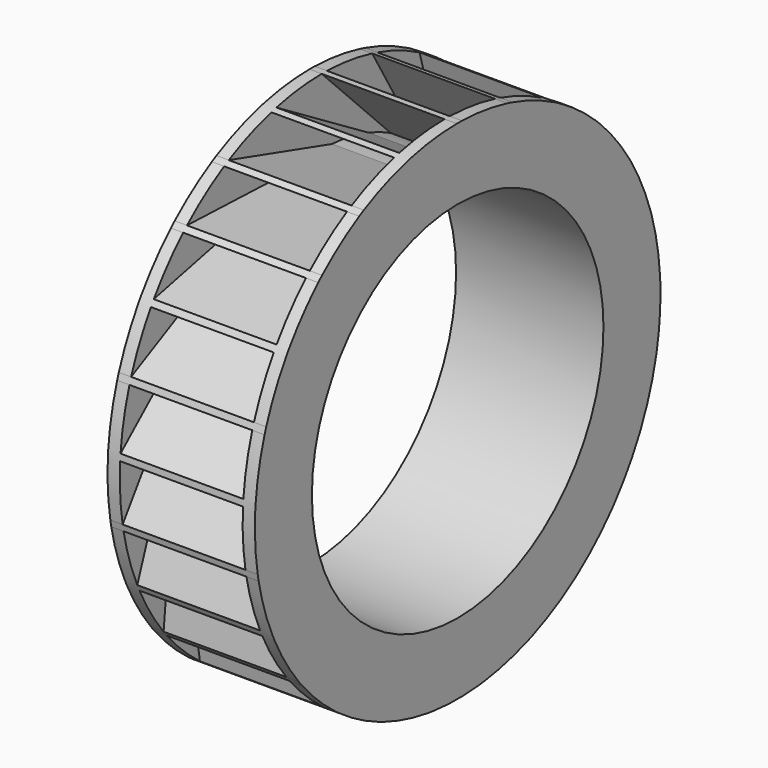
from build123d import *

# Parameters (mm, degrees)
F1_DEPTH      = 44
F1_DEPTH_BACK = 4
F2_DEPTH      = 40


with BuildPart() as f1:
    # F0 (on Right) → F1 (new body, two sides)
    with BuildSketch(Plane.YZ) as f1_sk:
        with BuildLine():
            Line((47.9947331255, -37.3985428132), (81.1532544526, -15.1212364493))
            ThreePointArc((81.1532544526, -15.1212364493), (82.2000719436, -7.5928039926), (82.55, 0))
            ThreePointArc((82.55, 0), (82.5323765572, 1.7056728359), (82.4795137535, 3.41061739))
            Line((82.4795137535, 3.41061739), (53.3191059714, -29.3124265585))
            ThreePointArc((53.3191059714, -29.3124265585), (50.81800682, -33.4615539863), (47.9947331255, -37.3985428132))
        make_face()
        with BuildLine():
            ThreePointArc((80.7364542136, -17.2083543957), (80.9515809502, -16.166138737), (81.1532544526, -15.1212364493))
            Line((81.1532544526, -15.1212364493), (47.9947331255, -37.3985428132))
            ThreePointArc((47.9947331255, -37.3985428132), (46.2234468965, -39.5668847567), (44.354284157, -41.6514452242))
            Line((44.354284157, -41.6514452242), (80.7364542136, -17.2083543957))
        make_face()
        with BuildLine():
            ThreePointArc((74.8431771472, -34.8281686931), (78.2870991132, -26.1845873071), (80.7364542136, -17.2083543957))
            Line((80.7364542136, -17.2083543957), (44.354284157, -41.6514452242))
            ThreePointArc((44.354284157, -41.6514452242), (40.8999156028, -45.0482221184), (37.1862509359, -48.1594035851))
            Line((37.1862509359, -48.1594035851), (74.8431771472, -34.8281686931))
        make_face()
        with BuildLine():
            ThreePointArc((44.354284157, -41.6514452242), (46.2234468965, -39.5668847567), (47.9947331255, -37.3985428132))
            ThreePointArc((47.9947331255, -37.3985428132), (50.81800682, -33.4615539863), (53.3191059714, -29.3124265585))
            ThreePointArc((53.3191059714, -29.3124265585), (54.6111364189, -26.8285145206), (55.7875297206, -24.2877940541))
            ThreePointArc((55.7875297206, -24.2877940541), (57.5430157732, -19.7723733543), (58.9336922637, -15.1316003287))
            ThreePointArc((58.9336922637, -15.1316003287), (59.5674073943, -12.4044100488), (60.0749906511, -9.6509538703))
            ThreePointArc((60.0749906511, -9.6509538703), (60.652385417, -4.8408217868), (60.8452579281, 0))
            ThreePointArc((60.8452579281, 0), (60.7808390896, 2.7991091266), (60.5877189787, 5.5922912388))
            ThreePointArc((60.5877189787, 5.5922912388), (59.9507426211, 10.3948964169), (58.9336922637, 15.1316003287))
            ThreePointArc((58.9336922637, 15.1316003287), (58.1751871286, 17.8267499812), (57.2934980968, 20.4841521224))
            ThreePointArc((57.2934980968, 20.4841521224), (55.4821741829, 24.977465049), (53.3191059714, 29.3124265585))
            ThreePointArc((53.3191059714, 29.3124265585), (51.9141742069, 31.7342705722), (50.3993160187, 34.0889183928))
            ThreePointArc((50.3993160187, 34.0889183928), (47.5274566917, 37.9906076914), (44.354284157, 41.6514452242))
            ThreePointArc((44.354284157, 41.6514452242), (42.3912027929, 43.6478102327), (40.3383595594, 45.5517525502))
            ThreePointArc((40.3383595594, 45.5517525502), (36.5864143028, 48.6166607328), (32.6025195453, 51.3733504031))
            ThreePointArc((32.6025195453, 51.3733504031), (30.2046362034, 52.8187974509), (27.7427956149, 54.1524025673))
            ThreePointArc((27.7427956149, 54.1524025673), (23.3465129478, 56.1879501808), (18.8022187269, 57.8672790382))
            ThreePointArc((18.8022187269, 57.8672790382), (16.1202012364, 58.6709853713), (13.4040497911, 59.3504579724))
            ThreePointArc((13.4040497911, 59.3504579724), (8.6396643218, 60.2287440741), (3.8205053562, 60.7251937104))
            ThreePointArc((3.8205053562, 60.7251937104), (1.0228747397, 60.836659504), (-1.7769217777, 60.8193058275))
            ThreePointArc((-1.7769217777, 60.8193058275), (-6.610046188, 60.4851444715), (-11.4012644169, 59.7675211301))
            ThreePointArc((-11.4012644169, 59.7675211301), (-14.1387227387, 59.1797425785), (-16.8462428162, 58.4666530196))
            ThreePointArc((-16.8462428162, 58.4666530196), (-21.4444231857, 56.9410407928), (-25.9066508157, 55.0544353876))
            ThreePointArc((-25.9066508157, 55.0544353876), (-28.4119322689, 53.8043447789), (-30.8570524625, 52.4403253772))
            ThreePointArc((-30.8570524625, 52.4403253772), (-34.9313682076, 49.8191221067), (-38.7842270658, 46.8820769937))
            ThreePointArc((-38.7842270658, 46.8820769937), (-40.8999156028, 45.0482221184), (-42.9290000181, 43.1189792294))
            ThreePointArc((-42.9290000181, 43.1189792294), (-46.2234468965, 39.5668847567), (-49.224847691, 35.7639452821))
            ThreePointArc((-49.224847691, 35.7639452821), (-50.81800682, 33.4615539863), (-52.3035606209, 31.088309036))
            ThreePointArc((-52.3035606209, 31.088309036), (-54.6111364188, 26.8285145206), (-56.5724900994, 22.3986333578))
            ThreePointArc((-56.5724900994, 22.3986333578), (-57.5430157732, 19.7723733543), (-58.3916961508, 17.1042460511))
            ThreePointArc((-58.3916961508, 17.1042460511), (-59.5674073943, 12.4044100488), (-60.3654748958, 7.6259329232))
            ThreePointArc((-60.3654748958, 7.6259329232), (-60.652385417, 4.8408217868), (-60.8108666619, 2.0454603818))
            ThreePointArc((-60.8108666619, 2.0454603818), (-60.836659504, 1.0228747397), (-60.8452579281, 0))
            ThreePointArc((-60.8452579281, 0), (-60.7251937104, -3.8205053562), (-60.3654748958, -7.6259329232))
            ThreePointArc((-60.3654748958, -7.6259329232), (-59.9507426211, -10.3948964169), (-59.4090667739, -13.141849086))
            ThreePointArc((-59.4090667739, -13.141849086), (-58.1751871286, -17.8267499812), (-56.5724900994, -22.3986333578))
            ThreePointArc((-56.5724900994, -22.3986333578), (-55.4821741829, -24.977465049), (-54.2743767292, -27.5034078433))
            ThreePointArc((-54.2743767292, -27.5034078433), (-51.914174207, -31.7342705722), (-49.224847691, -35.7639452821))
            ThreePointArc((-49.224847691, -35.7639452821), (-47.5274566917, -37.9906076914), (-45.7294279875, -40.1368263354))
            ThreePointArc((-45.7294279875, -40.1368263354), (-42.3912027929, -43.6478102327), (-38.7842270658, -46.8820769937))
            ThreePointArc((-38.7842270658, -46.8820769937), (-36.5864143028, -48.6166607328), (-34.3111311042, -50.248300416))
            ThreePointArc((-34.3111311042, -50.248300416), (-30.2046362034, -52.8187974509), (-25.9066508157, -55.0544353876))
            ThreePointArc((-25.9066508157, -55.0544353876), (-23.3465129478, -56.1879501808), (-20.7369396661, -57.202488981))
            ThreePointArc((-20.7369396661, -57.202488981), (-16.1202012364, -58.6709853713), (-11.4012644169, -59.7675211301))
            ThreePointArc((-11.4012644169, -59.7675211301), (-8.6396643218, -60.2287440741), (-5.8597700437, -60.5624347874))
            ThreePointArc((-5.8597700437, -60.5624347874), (-1.0228747397, -60.836659504), (3.8205053562, -60.7251937104))
            ThreePointArc((3.8205053562, -60.7251937104), (6.610046188, -60.4851444715), (9.3855904813, -60.117020083))
            ThreePointArc((9.3855904813, -60.117020083), (14.1387227387, -59.1797425785), (18.8022187269, -57.8672790382))
            ThreePointArc((18.8022187269, -57.8672790382), (21.4444231857, -56.9410407928), (24.0412198385, -55.8942319118))
            ThreePointArc((24.0412198385, -55.8942319118), (28.4119322689, -53.8043447789), (32.6025195453, -51.3733504031))
            ThreePointArc((32.6025195453, -51.3733504031), (34.9313682076, -49.8191221067), (37.1862509359, -48.1594035851))
            ThreePointArc((37.1862509359, -48.1594035851), (40.8999156028, -45.0482221184), (44.354284157, -41.6514452242))
        make_face()
        with BuildLine():
            ThreePointArc((59.3452579281, 0), (0, -59.3452579281), (-59.3452579281, 0))
            ThreePointArc((-59.3452579281, 0), (0, 59.3452579281), (59.3452579281, 0))
        make_face(mode=Mode.SUBTRACT)
        with BuildLine():
            Line((53.3191059714, -29.3124265585), (82.4795137535, 3.41061739))
            ThreePointArc((82.4795137535, 3.41061739), (82.4286933935, 4.4735897712), (82.3641743199, 5.5358186926))
            Line((82.3641743199, 5.5358186926), (55.7875297206, -24.2877940541))
            ThreePointArc((55.7875297206, -24.2877940541), (54.6111364189, -26.8285145206), (53.3191059714, -29.3124265585))
        make_face()
        with BuildLine():
            ThreePointArc((73.9204263276, -36.7460619869), (74.3879829567, -35.7900892934), (74.8431771472, -34.8281686931))
            Line((74.8431771472, -34.8281686931), (37.1862509359, -48.1594035851))
            ThreePointArc((37.1862509359, -48.1594035851), (34.9313682076, -49.8191221067), (32.6025195453, -51.3733504031))
            Line((32.6025195453, -51.3733504031), (73.9204263276, -36.7460619869))
        make_face()
        with BuildLine():
            Line((55.7875297206, -24.2877940541), (82.3641743199, 5.5358186926))
            ThreePointArc((82.3641743199, 5.5358186926), (81.2180290542, 14.7693688612), (79.0400821059, 23.8152875418))
            Line((79.0400821059, 23.8152875418), (58.9336922637, -15.1316003287))
            ThreePointArc((58.9336922637, -15.1316003287), (57.5430157732, -19.7723733543), (55.7875297206, -24.2877940541))
        make_face()
        with BuildLine():
            ThreePointArc((63.8304277677, -52.3467190089), (69.3157238718, -44.8311601916), (73.9204263276, -36.7460619869))
            Line((73.9204263276, -36.7460619869), (32.6025195453, -51.3733504031))
            ThreePointArc((32.6025195453, -51.3733504031), (28.4119322689, -53.8043447789), (24.0412198385, -55.8942319118))
            Line((24.0412198385, -55.8942319118), (63.8304277677, -52.3467190089))
        make_face()
        with BuildLine():
            Line((58.9336922637, -15.1316003287), (79.0400821059, 23.8152875418))
            ThreePointArc((79.0400821059, 23.8152875418), (78.7265078793, 24.8322261814), (78.3998502005, 25.8450379868))
            Line((78.3998502005, 25.8450379868), (60.0749906511, -9.6509538703))
            ThreePointArc((60.0749906511, -9.6509538703), (59.5674073943, -12.4044100488), (58.9336922637, -15.1316003287))
        make_face()
        with BuildLine():
            ThreePointArc((62.4597061951, -53.9748793609), (63.1503144142, -53.1652169128), (63.8304277677, -52.3467190089))
            Line((63.8304277677, -52.3467190089), (24.0412198385, -55.8942319118))
            ThreePointArc((24.0412198385, -55.8942319118), (21.4444231857, -56.9410407928), (18.8022187269, -57.8672790382))
            Line((18.8022187269, -57.8672790382), (62.4597061951, -53.9748793609))
        make_face()
        with BuildLine():
            Line((60.0749906511, -9.6509538703), (78.3998502005, 25.8450379868))
            ThreePointArc((78.3998502005, 25.8450379868), (74.9934226463, 34.5034644607), (70.6342714104, 42.7235555908))
            Line((70.6342714104, 42.7235555908), (60.8452579281, 0))
            ThreePointArc((60.8452579281, 0), (60.652385417, -4.8408217868), (60.0749906511, -9.6509538703))
        make_face()
        with BuildLine():
            ThreePointArc((48.8069778596, -66.5761324516), (55.9889867741, -60.6608264039), (62.4597061951, -53.9748793609))
            Line((62.4597061951, -53.9748793609), (18.8022187269, -57.8672790382))
            ThreePointArc((18.8022187269, -57.8672790382), (14.1387227387, -59.1797425785), (9.3855904813, -60.117020083))
            Line((9.3855904813, -60.117020083), (48.8069778596, -66.5761324516))
        make_face()
        with BuildLine():
            Line((60.8452579281, 0), (70.6342714104, 42.7235555908))
            ThreePointArc((70.6342714104, 42.7235555908), (70.0776463393, 43.630562494), (69.5093751585, 44.5303184928))
            Line((69.5093751585, 44.5303184928), (60.5877189787, 5.5922912388))
            ThreePointArc((60.5877189787, 5.5922912388), (60.7808390896, 2.7991091266), (60.8452579281, 0))
        make_face()
        with BuildLine():
            ThreePointArc((47.0744130116, -67.8122565589), (47.9446793664, -67.1997784256), (48.8069778596, -66.5761324516))
            Line((48.8069778596, -66.5761324516), (9.3855904813, -60.117020083))
            ThreePointArc((9.3855904813, -60.117020083), (6.610046188, -60.4851444715), (3.8205053562, -60.7251937104))
            Line((3.8205053562, -60.7251937104), (47.0744130116, -67.8122565589))
        make_face()
        with BuildLine():
            Line((60.5877189787, 5.5922912388), (69.5093751585, 44.5303184928))
            ThreePointArc((69.5093751585, 44.5303184928), (64.0567036871, 52.0695804932), (57.7902496675, 58.9473455159))
            Line((57.7902496675, 58.9473455159), (58.9336922637, 15.1316003287))
            ThreePointArc((58.9336922637, 15.1316003287), (59.9507426211, 10.3948964169), (60.5877189787, 5.5922912388))
        make_face()
        with BuildLine():
            ThreePointArc((30.7168060331, -76.6223226424), (39.1442557244, -72.6789497983), (47.0744130116, -67.8122565589))
            Line((47.0744130116, -67.8122565589), (3.8205053562, -60.7251937104))
            ThreePointArc((3.8205053562, -60.7251937104), (-1.0228747397, -60.836659504), (-5.8597700437, -60.5624347874))
            Line((-5.8597700437, -60.5624347874), (30.7168060331, -76.6223226424))
        make_face()
        with BuildLine():
            Line((58.9336922637, 15.1316003287), (57.7902496675, 58.9473455159))
            ThreePointArc((57.7902496675, 58.9473455159), (57.0255485522, 59.6874301032), (56.2513704377, 60.4175953169))
            Line((56.2513704377, 60.4175953169), (57.2934980968, 20.4841521224))
            ThreePointArc((57.2934980968, 20.4841521224), (58.1751871286, 17.8267499812), (58.9336922637, 15.1316003287))
        make_face()
        with BuildLine():
            ThreePointArc((28.731261331, -77.3887402813), (29.7265037859, -77.0119307164), (30.7168060331, -76.6223226424))
            Line((30.7168060331, -76.6223226424), (-5.8597700437, -60.5624347874))
            ThreePointArc((-5.8597700437, -60.5624347874), (-8.6396643218, -60.2287440741), (-11.4012644169, -59.7675211301))
            Line((-11.4012644169, -59.7675211301), (28.731261331, -77.3887402813))
        make_face()
        with BuildLine():
            Line((57.2934980968, 20.4841521224), (56.2513704377, 60.4175953169))
            ThreePointArc((56.2513704377, 60.4175953169), (49.0950664512, 66.3639732849), (41.3150540004, 71.4672569289))
            Line((41.3150540004, 71.4672569289), (53.3191059714, 29.3124265585))
            ThreePointArc((53.3191059714, 29.3124265585), (55.4821741829, 24.977465049), (57.2934980968, 20.4841521224))
        make_face()
        with BuildLine():
            ThreePointArc((10.6965843151, -81.8540505045), (19.8399471249, -80.1303874824), (28.731261331, -77.3887402813))
            Line((28.731261331, -77.3887402813), (-11.4012644169, -59.7675211301))
            ThreePointArc((-11.4012644169, -59.7675211301), (-16.1202012364, -58.6709853713), (-20.7369396661, -57.202488981))
            Line((-20.7369396661, -57.202488981), (10.6965843151, -81.8540505045))
        make_face()
        with BuildLine():
            Line((53.3191059714, 29.3124265585), (41.3150540004, 71.4672569289))
            ThreePointArc((41.3150540004, 71.4672569289), (40.3903258242, 71.9939169639), (39.4588852343, 72.5086124269))
            Line((39.4588852343, 72.5086124269), (50.3993160187, 34.0889183928))
            ThreePointArc((50.3993160187, 34.0889183928), (51.9141742069, 31.7342705722), (53.3191059714, 29.3124265585))
        make_face()
        with BuildLine():
            ThreePointArc((8.5828188348, -82.102604836), (9.640502646, -81.9851401702), (10.6965843151, -81.8540505045))
            Line((10.6965843151, -81.8540505045), (-20.7369396661, -57.202488981))
            ThreePointArc((-20.7369396661, -57.202488981), (-23.3465129478, -56.1879501808), (-25.9066508157, -55.0544353876))
            Line((-25.9066508157, -55.0544353876), (8.5828188348, -82.102604836))
        make_face()
        with BuildLine():
            Line((50.3993160187, 34.0889183928), (39.4588852343, 72.5086124269))
            ThreePointArc((39.4588852343, 72.5086124269), (31.0486056311, 76.4884735654), (22.2438815442, 79.496617751))
            Line((22.2438815442, 79.496617751), (44.354284157, 41.6514452242))
            ThreePointArc((44.354284157, 41.6514452242), (47.5274566917, 37.9906076914), (50.3993160187, 34.0889183928))
        make_face()
        with BuildLine():
            ThreePointArc((-9.9957431348, -81.9425873352), (-0.7109783186, -82.546938222), (8.5828188348, -82.102604836))
            Line((8.5828188348, -82.102604836), (-25.9066508157, -55.0544353876))
            ThreePointArc((-25.9066508157, -55.0544353876), (-30.2046362034, -52.8187974509), (-34.3111311042, -50.248300416))
            Line((-34.3111311042, -50.248300416), (-9.9957431348, -81.9425873352))
        make_face()
        with BuildLine():
            Line((44.354284157, 41.6514452242), (22.2438815442, 79.496617751))
            ThreePointArc((22.2438815442, 79.496617751), (21.2172303795, 79.7767612468), (20.1870531519, 80.04364675))
            Line((20.1870531519, 80.04364675), (40.3383595594, 45.5517525502))
            ThreePointArc((40.3383595594, 45.5517525502), (42.3912027929, 43.6478102327), (44.354284157, 41.6514452242))
        make_face()
        with BuildLine():
            ThreePointArc((-12.1049137342, -81.6576607765), (-11.0512467304, -81.8069217469), (-9.9957431348, -81.9425873352))
            Line((-9.9957431348, -81.9425873352), (-34.3111311042, -50.248300416))
            ThreePointArc((-34.3111311042, -50.248300416), (-36.5864143028, -48.6166607328), (-38.7842270658, -46.8820769937))
            Line((-38.7842270658, -46.8820769937), (-12.1049137342, -81.6576607765))
        make_face()
        with BuildLine():
            Line((40.3383595594, 45.5517525502), (20.1870531519, 80.04364675))
            ThreePointArc((20.1870531519, 80.04364675), (11.0512467304, 81.8069217469), (1.7750442034, 82.5309137116))
            Line((1.7750442034, 82.5309137116), (32.6025195453, 51.3733504031))
            ThreePointArc((32.6025195453, 51.3733504031), (36.5864143028, 48.6166607328), (40.3383595594, 45.5517525502))
        make_face()
        with BuildLine():
            ThreePointArc((-30.0600012817, -76.8823700399), (-21.2172303795, -79.7767612468), (-12.1049137342, -81.6576607765))
            Line((-12.1049137342, -81.6576607765), (-38.7842270658, -46.8820769937))
            ThreePointArc((-38.7842270658, -46.8820769937), (-42.3912027929, -43.6478102327), (-45.7294279875, -40.1368263354))
            Line((-45.7294279875, -40.1368263354), (-30.0600012817, -76.8823700399))
        make_face()
        with BuildLine():
            Line((32.6025195453, 51.3733504031), (1.7750442034, 82.5309137116))
            ThreePointArc((1.7750442034, 82.5309137116), (0.7109783186, 82.546938222), (-0.3532057228, 82.5492443679))
            Line((-0.3532057228, 82.5492443679), (27.7427956149, 54.1524025673))
            ThreePointArc((27.7427956149, 54.1524025673), (30.2046362034, 52.8187974509), (32.6025195453, 51.3733504031))
        make_face()
        with BuildLine():
            ThreePointArc((-32.0320500545, -76.0818655746), (-31.0486056311, -76.4884735654), (-30.0600012817, -76.8823700399))
            Line((-30.0600012817, -76.8823700399), (-45.7294279875, -40.1368263354))
            ThreePointArc((-45.7294279875, -40.1368263354), (-47.5274566917, -37.9906076914), (-49.224847691, -35.7639452821))
            Line((-49.224847691, -35.7639452821), (-32.0320500545, -76.0818655746))
        make_face()
        with BuildLine():
            Line((27.7427956149, 54.1524025673), (-0.3532057228, 82.5492443679))
            ThreePointArc((-0.3532057228, 82.5492443679), (-9.640502646, 81.9851401702), (-18.8053256929, 80.3794888363))
            Line((-18.8053256929, 80.3794888363), (18.8022187269, 57.8672790382))
            ThreePointArc((18.8022187269, 57.8672790382), (23.3465129478, 56.1879501808), (27.7427956149, 54.1524025673))
        make_face()
        with BuildLine():
            ThreePointArc((-48.2354789951, -66.9913506814), (-40.3903258242, -71.9939169639), (-32.0320500545, -76.0818655746))
            Line((-32.0320500545, -76.0818655746), (-49.224847691, -35.7639452821))
            ThreePointArc((-49.224847691, -35.7639452821), (-51.914174207, -31.7342705722), (-54.2743767292, -27.5034078433))
            Line((-54.2743767292, -27.5034078433), (-48.2354789951, -66.9913506814))
        make_face()
        with BuildLine():
            Line((18.8022187269, 57.8672790382), (-18.8053256929, 80.3794888363))
            ThreePointArc((-18.8053256929, 80.3794888363), (-19.8399471249, 80.1303874824), (-20.8712713829, 79.8679693673))
            Line((-20.8712713829, 79.8679693673), (13.4040497911, 59.3504579724))
            ThreePointArc((13.4040497911, 59.3504579724), (16.1202012364, 58.6709853713), (18.8022187269, 57.8672790382))
        make_face()
        with BuildLine():
            ThreePointArc((-49.9464948643, -65.7255669491), (-49.0950664512, -66.3639732849), (-48.2354789951, -66.9913506814))
            Line((-48.2354789951, -66.9913506814), (-54.2743767292, -27.5034078433))
            ThreePointArc((-54.2743767292, -27.5034078433), (-55.4821741829, -24.977465049), (-56.5724900994, -22.3986333578))
            Line((-56.5724900994, -22.3986333578), (-49.9464948643, -65.7255669491))
        make_face()
        with BuildLine():
            Line((13.4040497911, 59.3504579724), (-20.8712713829, 79.8679693673))
            ThreePointArc((-20.8712713829, 79.8679693673), (-29.7265037859, 77.0119307164), (-38.2040878147, 73.1775250623))
            Line((-38.2040878147, 73.1775250623), (3.8205053562, 60.7251937104))
            ThreePointArc((3.8205053562, 60.7251937104), (8.6396643218, 60.2287440741), (13.4040497911, 59.3504579724))
        make_face()
        with BuildLine():
            ThreePointArc((-63.3801441656, -52.8910183826), (-57.0255485522, -59.6874301032), (-49.9464948643, -65.7255669491))
            Line((-49.9464948643, -65.7255669491), (-56.5724900994, -22.3986333578))
            ThreePointArc((-56.5724900994, -22.3986333578), (-58.1751871286, -17.8267499812), (-59.4090667739, -13.141849086))
            Line((-59.4090667739, -13.141849086), (-63.3801441656, -52.8910183826))
        make_face()
        with BuildLine():
            Line((3.8205053562, 60.7251937104), (-38.2040878147, 73.1775250623))
            ThreePointArc((-38.2040878147, 73.1775250623), (-39.1442557244, 72.6789497983), (-40.0779183029, 72.1682961175))
            Line((-40.0779183029, 72.1682961175), (-1.7769217777, 60.8193058275))
            ThreePointArc((-1.7769217777, 60.8193058275), (1.0228747397, 60.836659504), (3.8205053562, 60.7251937104))
        make_face()
        with BuildLine():
            ThreePointArc((-64.7226177113, -51.2394892304), (-64.0567036871, -52.0695804932), (-63.3801441656, -52.8910183826))
            Line((-63.3801441656, -52.8910183826), (-59.4090667739, -13.141849086))
            ThreePointArc((-59.4090667739, -13.141849086), (-59.9507426211, -10.3948964169), (-60.3654748958, -7.6259329232))
            Line((-60.3654748958, -7.6259329232), (-64.7226177113, -51.2394892304))
        make_face()
        with BuildLine():
            Line((-1.7769217777, 60.8193058275), (-40.0779183029, 72.1682961175))
            ThreePointArc((-40.0779183029, 72.1682961175), (-47.9446793664, 67.1997784256), (-55.2023465944, 61.3775482605))
            Line((-55.2023465944, 61.3775482605), (-11.4012644169, 59.7675211301))
            ThreePointArc((-11.4012644169, 59.7675211301), (-6.610046188, 60.4851444715), (-1.7769217777, 60.8193058275))
        make_face()
        with BuildLine():
            ThreePointArc((-74.5424017823, -35.4673488793), (-70.0776463393, -43.630562494), (-64.7226177113, -51.2394892304))
            Line((-64.7226177113, -51.2394892304), (-60.3654748958, -7.6259329232))
            ThreePointArc((-60.3654748958, -7.6259329232), (-60.7251937104, -3.8205053562), (-60.8452579281, 0))
            ThreePointArc((-60.8452579281, 0), (-60.836659504, 1.0228747397), (-60.8108666619, 2.0454603818))
            Line((-60.8108666619, 2.0454603818), (-74.5424017823, -35.4673488793))
        make_face()
        with BuildLine():
            Line((-11.4012644169, 59.7675211301), (-55.2023465944, 61.3775482605))
            ThreePointArc((-55.2023465944, 61.3775482605), (-55.9889867741, 60.6608264039), (-56.7663222196, 59.9340234062))
            Line((-56.7663222196, 59.9340234062), (-16.8462428162, 58.4666530196))
            ThreePointArc((-16.8462428162, 58.4666530196), (-14.1387227387, 59.1797425785), (-11.4012644169, 59.7675211301))
        make_face()
        with BuildLine():
            ThreePointArc((-75.4319804544, -33.5338459578), (-74.9934226463, -34.5034644607), (-74.5424017823, -35.4673488793))
            Line((-74.5424017823, -35.4673488793), (-60.8108666619, 2.0454603818))
            ThreePointArc((-60.8108666619, 2.0454603818), (-60.652385417, 4.8408217868), (-60.3654748958, 7.6259329232))
            Line((-60.3654748958, 7.6259329232), (-75.4319804544, -33.5338459578))
        make_face()
        with BuildLine():
            Line((-16.8462428162, 58.4666530196), (-56.7663222196, 59.9340234062))
            ThreePointArc((-56.7663222196, 59.9340234062), (-63.1503144142, 53.1652169128), (-68.7320389175, 45.7209943707))
            Line((-68.7320389175, 45.7209943707), (-25.9066508157, 55.0544353876))
            ThreePointArc((-25.9066508157, 55.0544353876), (-21.4444231857, 56.9410407928), (-16.8462428162, 58.4666530196))
        make_face()
        with BuildLine():
            ThreePointArc((-81.0208861473, -15.8151354061), (-78.7265078793, -24.8322261814), (-75.4319804544, -33.5338459578))
            Line((-75.4319804544, -33.5338459578), (-60.3654748958, 7.6259329232))
            ThreePointArc((-60.3654748958, 7.6259329232), (-59.5674073943, 12.4044100488), (-58.3916961508, 17.1042460511))
            Line((-58.3916961508, 17.1042460511), (-81.0208861473, -15.8151354061))
        make_face()
        with BuildLine():
            Line((-25.9066508157, 55.0544353876), (-68.7320389175, 45.7209943707))
            ThreePointArc((-68.7320389175, 45.7209943707), (-69.3157238718, 44.8311601916), (-69.8878893393, 43.9338755824))
            Line((-69.8878893393, 43.9338755824), (-30.8570524625, 52.4403253772))
            ThreePointArc((-30.8570524625, 52.4403253772), (-28.4119322689, 53.8043447789), (-25.9066508157, 55.0544353876))
        make_face()
        with BuildLine():
            ThreePointArc((-81.4016744462, -13.7211478147), (-81.2180290542, -14.7693688612), (-81.0208861473, -15.8151354061))
            Line((-81.0208861473, -15.8151354061), (-58.3916961508, 17.1042460511))
            ThreePointArc((-58.3916961508, 17.1042460511), (-57.5430157732, 19.7723733543), (-56.5724900994, 22.3986333578))
            Line((-56.5724900994, 22.3986333578), (-81.4016744462, -13.7211478147))
        make_face()
        with BuildLine():
            Line((-30.8570524625, 52.4403253772), (-69.8878893393, 43.9338755824))
            ThreePointArc((-69.8878893393, 43.9338755824), (-74.3879829567, 35.7900892934), (-77.9430444566, 27.1916222546))
            Line((-77.9430444566, 27.1916222546), (-38.7842270658, 46.8820769937))
            ThreePointArc((-38.7842270658, 46.8820769937), (-34.9313682076, 49.8191221067), (-30.8570524625, 52.4403253772))
        make_face()
        with BuildLine():
            ThreePointArc((-82.4085302616, 4.8308011886), (-82.4286933935, -4.4735897712), (-81.4016744462, -13.7211478147))
            Line((-81.4016744462, -13.7211478147), (-56.5724900994, 22.3986333578))
            ThreePointArc((-56.5724900994, 22.3986333578), (-54.6111364188, 26.8285145206), (-52.3035606209, 31.088309036))
            Line((-52.3035606209, 31.088309036), (-82.4085302616, 4.8308011886))
        make_face()
        with BuildLine():
            Line((-38.7842270658, 46.8820769937), (-77.9430444566, 27.1916222546))
            ThreePointArc((-77.9430444566, 27.1916222546), (-78.2870991132, 26.1845873071), (-78.6181433422, 25.1732007783))
            Line((-78.6181433422, 25.1732007783), (-42.9290000181, 43.1189792294))
            ThreePointArc((-42.9290000181, 43.1189792294), (-40.8999156028, 45.0482221184), (-38.7842270658, 46.8820769937))
        make_face()
        with BuildLine():
            ThreePointArc((-82.2566018581, 6.9537005083), (-82.3394079975, 5.8927405018), (-82.4085302616, 4.8308011886))
            Line((-82.4085302616, 4.8308011886), (-52.3035606209, 31.088309036))
            ThreePointArc((-52.3035606209, 31.088309036), (-50.81800682, 33.4615539863), (-49.224847691, 35.7639452821))
            Line((-49.224847691, 35.7639452821), (-82.2566018581, 6.9537005083))
        make_face()
        with BuildLine():
            Line((-42.9290000181, 43.1189792294), (-78.6181433422, 25.1732007783))
            ThreePointArc((-78.6181433422, 25.1732007783), (-80.9515809502, 16.166138737), (-82.2566018581, 6.9537005083))
            Line((-82.2566018581, 6.9537005083), (-49.224847691, 35.7639452821))
            ThreePointArc((-49.224847691, 35.7639452821), (-46.2234468965, 39.5668847567), (-42.9290000181, 43.1189792294))
        make_face()
    extrude(amount=F1_DEPTH)
    extrude(f1_sk.sketch, amount=-F1_DEPTH_BACK)

    # F0 (on Right) → F2 (cut)
    with BuildSketch(Plane.YZ):
        with BuildLine():
            Line((47.9947331255, -37.3985428132), (81.1532544526, -15.1212364493))
            ThreePointArc((81.1532544526, -15.1212364493), (82.2000719436, -7.5928039926), (82.55, 0))
            ThreePointArc((82.55, 0), (82.5323765572, 1.7056728359), (82.4795137535, 3.41061739))
            Line((82.4795137535, 3.41061739), (53.3191059714, -29.3124265585))
            ThreePointArc((53.3191059714, -29.3124265585), (50.81800682, -33.4615539863), (47.9947331255, -37.3985428132))
        make_face()
        with BuildLine():
            ThreePointArc((74.8431771472, -34.8281686931), (78.2870991132, -26.1845873071), (80.7364542136, -17.2083543957))
            Line((80.7364542136, -17.2083543957), (44.354284157, -41.6514452242))
            ThreePointArc((44.354284157, -41.6514452242), (40.8999156028, -45.0482221184), (37.1862509359, -48.1594035851))
            Line((37.1862509359, -48.1594035851), (74.8431771472, -34.8281686931))
        make_face()
        with BuildLine():
            Line((55.7875297206, -24.2877940541), (82.3641743199, 5.5358186926))
            ThreePointArc((82.3641743199, 5.5358186926), (81.2180290542, 14.7693688612), (79.0400821059, 23.8152875418))
            Line((79.0400821059, 23.8152875418), (58.9336922637, -15.1316003287))
            ThreePointArc((58.9336922637, -15.1316003287), (57.5430157732, -19.7723733543), (55.7875297206, -24.2877940541))
        make_face()
        with BuildLine():
            ThreePointArc((63.8304277677, -52.3467190089), (69.3157238718, -44.8311601916), (73.9204263276, -36.7460619869))
            Line((73.9204263276, -36.7460619869), (32.6025195453, -51.3733504031))
            ThreePointArc((32.6025195453, -51.3733504031), (28.4119322689, -53.8043447789), (24.0412198385, -55.8942319118))
            Line((24.0412198385, -55.8942319118), (63.8304277677, -52.3467190089))
        make_face()
        with BuildLine():
            Line((60.0749906511, -9.6509538703), (78.3998502005, 25.8450379868))
            ThreePointArc((78.3998502005, 25.8450379868), (74.9934226463, 34.5034644607), (70.6342714104, 42.7235555908))
            Line((70.6342714104, 42.7235555908), (60.8452579281, 0))
            ThreePointArc((60.8452579281, 0), (60.652385417, -4.8408217868), (60.0749906511, -9.6509538703))
        make_face()
        with BuildLine():
            ThreePointArc((48.8069778596, -66.5761324516), (55.9889867741, -60.6608264039), (62.4597061951, -53.9748793609))
            Line((62.4597061951, -53.9748793609), (18.8022187269, -57.8672790382))
            ThreePointArc((18.8022187269, -57.8672790382), (14.1387227387, -59.1797425785), (9.3855904813, -60.117020083))
            Line((9.3855904813, -60.117020083), (48.8069778596, -66.5761324516))
        make_face()
        with BuildLine():
            Line((60.5877189787, 5.5922912388), (69.5093751585, 44.5303184928))
            ThreePointArc((69.5093751585, 44.5303184928), (64.0567036871, 52.0695804932), (57.7902496675, 58.9473455159))
            Line((57.7902496675, 58.9473455159), (58.9336922637, 15.1316003287))
            ThreePointArc((58.9336922637, 15.1316003287), (59.9507426211, 10.3948964169), (60.5877189787, 5.5922912388))
        make_face()
        with BuildLine():
            ThreePointArc((30.7168060331, -76.6223226424), (39.1442557244, -72.6789497983), (47.0744130116, -67.8122565589))
            Line((47.0744130116, -67.8122565589), (3.8205053562, -60.7251937104))
            ThreePointArc((3.8205053562, -60.7251937104), (-1.0228747397, -60.836659504), (-5.8597700437, -60.5624347874))
            Line((-5.8597700437, -60.5624347874), (30.7168060331, -76.6223226424))
        make_face()
        with BuildLine():
            Line((57.2934980968, 20.4841521224), (56.2513704377, 60.4175953169))
            ThreePointArc((56.2513704377, 60.4175953169), (49.0950664512, 66.3639732849), (41.3150540004, 71.4672569289))
            Line((41.3150540004, 71.4672569289), (53.3191059714, 29.3124265585))
            ThreePointArc((53.3191059714, 29.3124265585), (55.4821741829, 24.977465049), (57.2934980968, 20.4841521224))
        make_face()
        with BuildLine():
            ThreePointArc((10.6965843151, -81.8540505045), (19.8399471249, -80.1303874824), (28.731261331, -77.3887402813))
            Line((28.731261331, -77.3887402813), (-11.4012644169, -59.7675211301))
            ThreePointArc((-11.4012644169, -59.7675211301), (-16.1202012364, -58.6709853713), (-20.7369396661, -57.202488981))
            Line((-20.7369396661, -57.202488981), (10.6965843151, -81.8540505045))
        make_face()
        with BuildLine():
            Line((50.3993160187, 34.0889183928), (39.4588852343, 72.5086124269))
            ThreePointArc((39.4588852343, 72.5086124269), (31.0486056311, 76.4884735654), (22.2438815442, 79.496617751))
            Line((22.2438815442, 79.496617751), (44.354284157, 41.6514452242))
            ThreePointArc((44.354284157, 41.6514452242), (47.5274566917, 37.9906076914), (50.3993160187, 34.0889183928))
        make_face()
        with BuildLine():
            ThreePointArc((-9.9957431348, -81.9425873352), (-0.7109783186, -82.546938222), (8.5828188348, -82.102604836))
            Line((8.5828188348, -82.102604836), (-25.9066508157, -55.0544353876))
            ThreePointArc((-25.9066508157, -55.0544353876), (-30.2046362034, -52.8187974509), (-34.3111311042, -50.248300416))
            Line((-34.3111311042, -50.248300416), (-9.9957431348, -81.9425873352))
        make_face()
        with BuildLine():
            Line((40.3383595594, 45.5517525502), (20.1870531519, 80.04364675))
            ThreePointArc((20.1870531519, 80.04364675), (11.0512467304, 81.8069217469), (1.7750442034, 82.5309137116))
            Line((1.7750442034, 82.5309137116), (32.6025195453, 51.3733504031))
            ThreePointArc((32.6025195453, 51.3733504031), (36.5864143028, 48.6166607328), (40.3383595594, 45.5517525502))
        make_face()
        with BuildLine():
            ThreePointArc((-30.0600012817, -76.8823700399), (-21.2172303795, -79.7767612468), (-12.1049137342, -81.6576607765))
            Line((-12.1049137342, -81.6576607765), (-38.7842270658, -46.8820769937))
            ThreePointArc((-38.7842270658, -46.8820769937), (-42.3912027929, -43.6478102327), (-45.7294279875, -40.1368263354))
            Line((-45.7294279875, -40.1368263354), (-30.0600012817, -76.8823700399))
        make_face()
        with BuildLine():
            Line((27.7427956149, 54.1524025673), (-0.3532057228, 82.5492443679))
            ThreePointArc((-0.3532057228, 82.5492443679), (-9.640502646, 81.9851401702), (-18.8053256929, 80.3794888363))
            Line((-18.8053256929, 80.3794888363), (18.8022187269, 57.8672790382))
            ThreePointArc((18.8022187269, 57.8672790382), (23.3465129478, 56.1879501808), (27.7427956149, 54.1524025673))
        make_face()
        with BuildLine():
            ThreePointArc((-48.2354789951, -66.9913506814), (-40.3903258242, -71.9939169639), (-32.0320500545, -76.0818655746))
            Line((-32.0320500545, -76.0818655746), (-49.224847691, -35.7639452821))
            ThreePointArc((-49.224847691, -35.7639452821), (-51.914174207, -31.7342705722), (-54.2743767292, -27.5034078433))
            Line((-54.2743767292, -27.5034078433), (-48.2354789951, -66.9913506814))
        make_face()
        with BuildLine():
            Line((13.4040497911, 59.3504579724), (-20.8712713829, 79.8679693673))
            ThreePointArc((-20.8712713829, 79.8679693673), (-29.7265037859, 77.0119307164), (-38.2040878147, 73.1775250623))
            Line((-38.2040878147, 73.1775250623), (3.8205053562, 60.7251937104))
            ThreePointArc((3.8205053562, 60.7251937104), (8.6396643218, 60.2287440741), (13.4040497911, 59.3504579724))
        make_face()
        with BuildLine():
            ThreePointArc((-63.3801441656, -52.8910183826), (-57.0255485522, -59.6874301032), (-49.9464948643, -65.7255669491))
            Line((-49.9464948643, -65.7255669491), (-56.5724900994, -22.3986333578))
            ThreePointArc((-56.5724900994, -22.3986333578), (-58.1751871286, -17.8267499812), (-59.4090667739, -13.141849086))
            Line((-59.4090667739, -13.141849086), (-63.3801441656, -52.8910183826))
        make_face()
        with BuildLine():
            Line((-1.7769217777, 60.8193058275), (-40.0779183029, 72.1682961175))
            ThreePointArc((-40.0779183029, 72.1682961175), (-47.9446793664, 67.1997784256), (-55.2023465944, 61.3775482605))
            Line((-55.2023465944, 61.3775482605), (-11.4012644169, 59.7675211301))
            ThreePointArc((-11.4012644169, 59.7675211301), (-6.610046188, 60.4851444715), (-1.7769217777, 60.8193058275))
        make_face()
        with BuildLine():
            ThreePointArc((-74.5424017823, -35.4673488793), (-70.0776463393, -43.630562494), (-64.7226177113, -51.2394892304))
            Line((-64.7226177113, -51.2394892304), (-60.3654748958, -7.6259329232))
            ThreePointArc((-60.3654748958, -7.6259329232), (-60.7251937104, -3.8205053562), (-60.8452579281, 0))
            ThreePointArc((-60.8452579281, 0), (-60.836659504, 1.0228747397), (-60.8108666619, 2.0454603818))
            Line((-60.8108666619, 2.0454603818), (-74.5424017823, -35.4673488793))
        make_face()
        with BuildLine():
            Line((-16.8462428162, 58.4666530196), (-56.7663222196, 59.9340234062))
            ThreePointArc((-56.7663222196, 59.9340234062), (-63.1503144142, 53.1652169128), (-68.7320389175, 45.7209943707))
            Line((-68.7320389175, 45.7209943707), (-25.9066508157, 55.0544353876))
            ThreePointArc((-25.9066508157, 55.0544353876), (-21.4444231857, 56.9410407928), (-16.8462428162, 58.4666530196))
        make_face()
        with BuildLine():
            ThreePointArc((-81.0208861473, -15.8151354061), (-78.7265078793, -24.8322261814), (-75.4319804544, -33.5338459578))
            Line((-75.4319804544, -33.5338459578), (-60.3654748958, 7.6259329232))
            ThreePointArc((-60.3654748958, 7.6259329232), (-59.5674073943, 12.4044100488), (-58.3916961508, 17.1042460511))
            Line((-58.3916961508, 17.1042460511), (-81.0208861473, -15.8151354061))
        make_face()
        with BuildLine():
            Line((-30.8570524625, 52.4403253772), (-69.8878893393, 43.9338755824))
            ThreePointArc((-69.8878893393, 43.9338755824), (-74.3879829567, 35.7900892934), (-77.9430444566, 27.1916222546))
            Line((-77.9430444566, 27.1916222546), (-38.7842270658, 46.8820769937))
            ThreePointArc((-38.7842270658, 46.8820769937), (-34.9313682076, 49.8191221067), (-30.8570524625, 52.4403253772))
        make_face()
        with BuildLine():
            ThreePointArc((-82.4085302616, 4.8308011886), (-82.4286933935, -4.4735897712), (-81.4016744462, -13.7211478147))
            Line((-81.4016744462, -13.7211478147), (-56.5724900994, 22.3986333578))
            ThreePointArc((-56.5724900994, 22.3986333578), (-54.6111364188, 26.8285145206), (-52.3035606209, 31.088309036))
            Line((-52.3035606209, 31.088309036), (-82.4085302616, 4.8308011886))
        make_face()
        with BuildLine():
            Line((-42.9290000181, 43.1189792294), (-78.6181433422, 25.1732007783))
            ThreePointArc((-78.6181433422, 25.1732007783), (-80.9515809502, 16.166138737), (-82.2566018581, 6.9537005083))
            Line((-82.2566018581, 6.9537005083), (-49.224847691, 35.7639452821))
            ThreePointArc((-49.224847691, 35.7639452821), (-46.2234468965, 39.5668847567), (-42.9290000181, 43.1189792294))
        make_face()
    extrude(amount=F2_DEPTH, mode=Mode.SUBTRACT)


solid = f1.part
